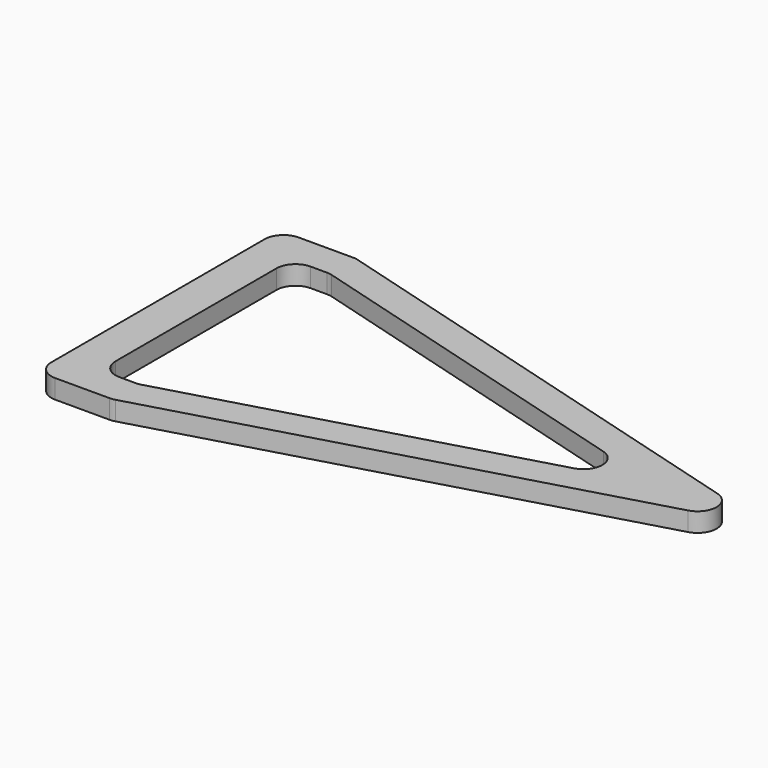
from build123d import *

# Parameters (mm, degrees)
F1_DEPTH = 6.35
F2_W     = 12.7
F2_H     = 79.8285714286
F3_DEPTH = 6.35
F4_R     = 6.35
F5_R     = 6.35


with BuildPart() as f1:
    # F0 (on Top) → F1 (new body)
    with BuildSketch(Plane.XY):
        Polygon((-177.8, 0), (0, 0), (-177.8, 50.8), align=None)
        Polygon((-177.8, -50.8), (0, 0), (-177.8, 0), align=None)
        Polygon((-177.8, 0), (-177.8, 50.8), (-203.2, 50.8), (-203.2, -50.8), (-177.8, -50.8), align=None)
    extrude(amount=F1_DEPTH)

    # F2 (on face) → F3 (cut, through all)
    with BuildSketch(Plane.XY.offset(6.35)):
        Polygon((-177.8, 39.9142857143), (-177.8, -39.9142857143), (-38.1, 0), align=None)
        with Locations((-184.15, 0)):
            Rectangle(F2_W, F2_H)
    extrude(amount=-F3_DEPTH, mode=Mode.SUBTRACT)

    # F4
    f4_edges = [f1.edges().sort_by_distance(p)[0] for p in [
        (-177.8, -50.8, 3.175),
        (-177.8, 50.8, 3.175),
        (-203.2, -50.8, 3.175),
        (-203.2, 50.8, 3.175),
    ]]
    fillet(f4_edges, radius=F4_R)

    # F5
    f5_edges = [f1.edges().sort_by_distance(p)[0] for p in [
        (-177.8, -39.914286, 3.175),
        (-190.5, -39.914286, 3.175),
        (-190.5, 39.914286, 3.175),
        (-177.8, 39.914286, 3.175),
        (0, 0, 3.175),
        (-38.1, 0, 3.175),
    ]]
    fillet(f5_edges, radius=F5_R)


solid = f1.part
